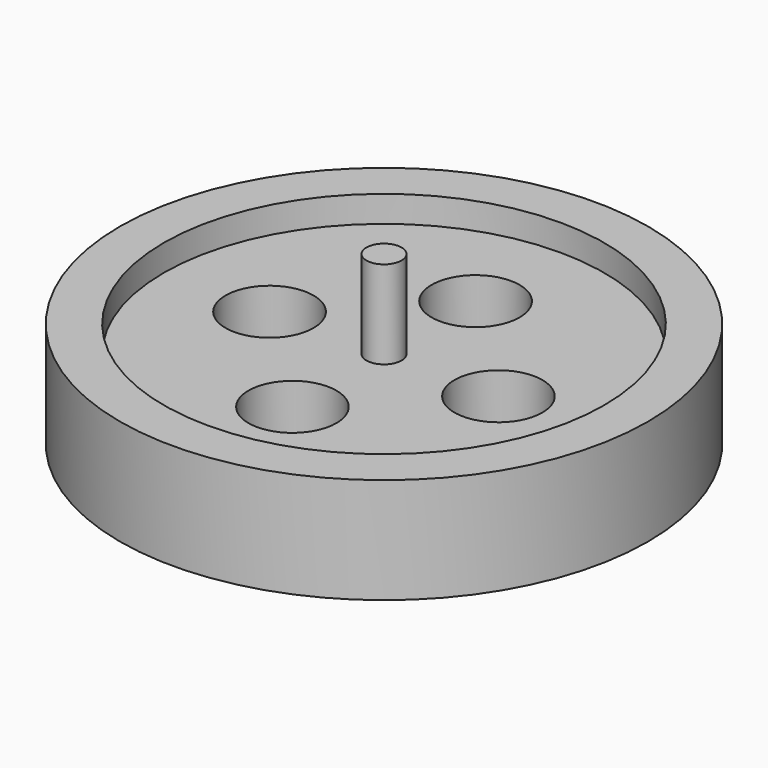
from build123d import *

# Parameters (mm, degrees)
F0_R     = 38.1
F1_DEPTH = 15.24
F2_R     = 31.75
F3_DEPTH = 3.81
F4_R     = 31.75
F5_DEPTH = 3.81
F6_R     = 6.35
F7_DEPTH = 11.431
F8_W     = 2.54
F8_H     = 12.7


# Not quite as in the source:
# - a feature names something its author has since deleted; it is built from what else it names


with BuildPart() as f1:
    # F0 (on Top) → F1 (new body)
    with BuildSketch(Plane.XY):
        Circle(F0_R)
    extrude(amount=F1_DEPTH)

    # F2 (on face) → F3 (cut)
    with BuildSketch(Plane.XY.offset(15.24)):
        Circle(F2_R)
    extrude(amount=-F3_DEPTH, mode=Mode.SUBTRACT)

    # F4 (on face) → F5 (cut)
    with BuildSketch(Plane(origin=(0, 0, 0), x_dir=(1, 0, 0), z_dir=(0, 0, -1))):
        Circle(F4_R)
    extrude(amount=-F5_DEPTH, mode=Mode.SUBTRACT)

    # F6 (on face) → F7 (cut, through all)
    with BuildSketch(Plane.XY.offset(11.43)):
        with Locations((0, 16.51)):
            Circle(F6_R)
        with Locations((16.51, 0)):
            Circle(F6_R)
        with Locations((0, -16.51)):
            Circle(F6_R)
        with Locations((-16.51, 0)):
            Circle(F6_R)
    extrude(amount=-F7_DEPTH, mode=Mode.SUBTRACT)

    # F8 (on Front) → F10 (revolve)
    with BuildSketch(Plane.XZ):
        with Locations((1.27, 17.78)):
            Rectangle(F8_W, F8_H)
    revolve(axis=Axis((0, 0, 19.05), (0, 0, -1)))


solid = f1.part
